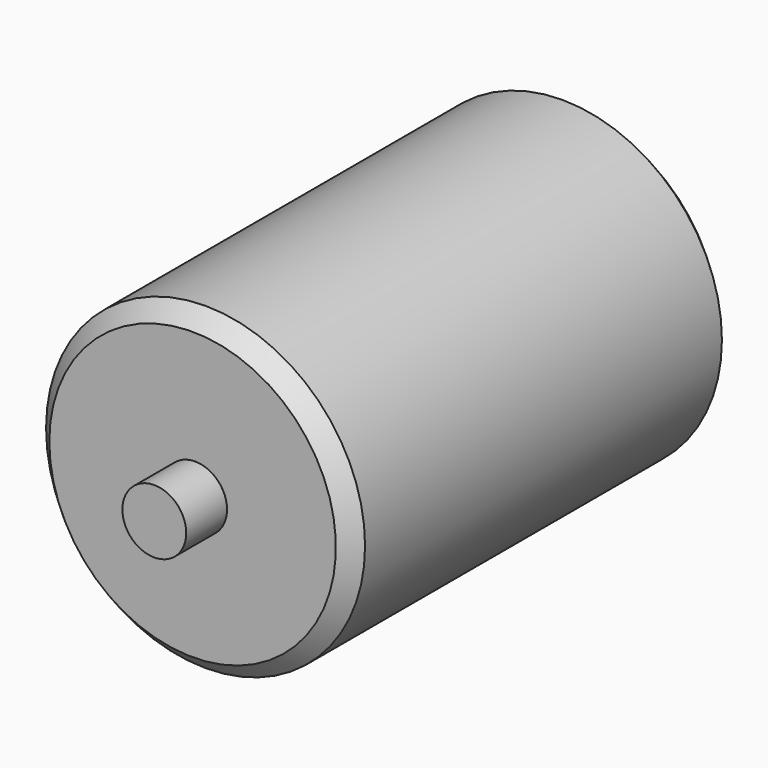
from build123d import *

# Parameters (mm, degrees)
F0_R     = 10
F1_DEPTH = 16
F2_R     = 50
F2_R_2   = 10
F3_DEPTH = 150
F6_DEPTH = 16
F7_SIZE  = 5.08


with BuildPart() as f1:
    # F0 (on Front) → F1 (new body)
    with BuildSketch(Plane.XZ):
        with Locations((0.7890519919, -0.6312426412)):
            Circle(F0_R)
    extrude(amount=F1_DEPTH)


with BuildPart() as f3:
    # F2 (on face) → F3 (new body)
    with BuildSketch(Plane(origin=(0, 0, 0), x_dir=(-1, 0, 0), z_dir=(0, 1, 0))):
        Circle(F2_R)
        with Locations((-0.7890519919, -0.6312426412)):
            Circle(F2_R_2, mode=Mode.SUBTRACT)
    extrude(amount=F3_DEPTH)

    # F7
    f7_edges = [f3.edges().sort_by_distance(p)[0] for p in [
        (50, 150, 0),
        (50, 0, 0),
    ]]
    chamfer(f7_edges, length=F7_SIZE)


with BuildPart() as f6:
    # F5 (on face) → F6 (new body)
    with BuildSketch(Plane(origin=(0, 150, 0), x_dir=(-1, 0, 0), z_dir=(0, 1, 0))):
        with BuildLine():
            ThreePointArc((9.2109480081, -0.6312426412), (-4.099125069, 8.8050392655), (-8.5977352367, -6.8781991788))
            ThreePointArc((-8.5977352367, -6.8781991788), (2.5210210852, -10.067524548), (9.2109480081, -0.6312426412))
        make_face()
    extrude(amount=F6_DEPTH)


solid = Compound([f1.part, f3.part, f6.part])
